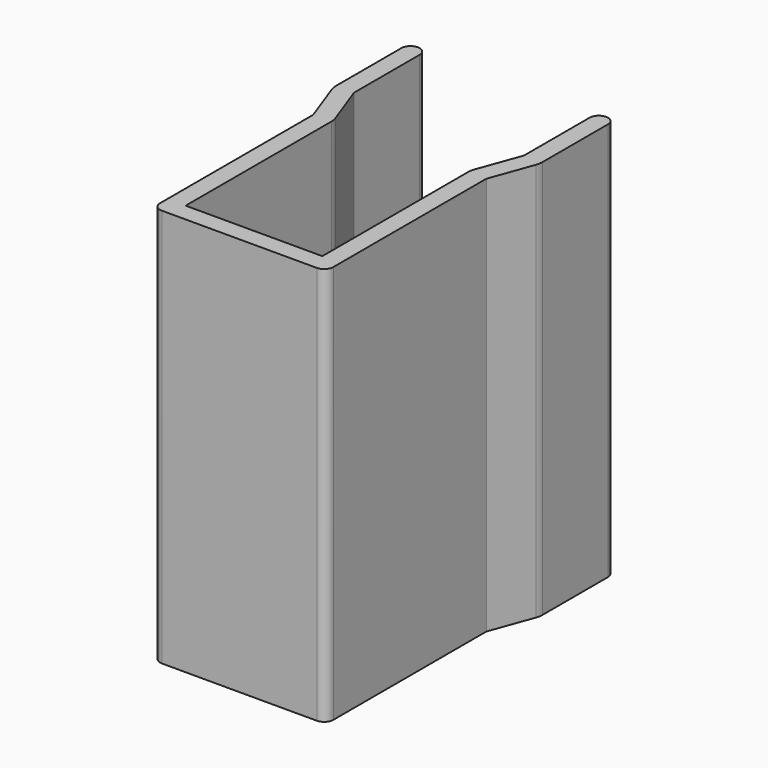
from build123d import *

# Parameters (mm, degrees)
F0_W     = 1.6
F0_H     = 8
F1_DEPTH = 35
F2_R     = 0.79999


# Not quite as in the source:
# - a fillet or chamfer is up to 0.001 mm smaller than in the source, because OpenCascade refuses the exact size


with BuildPart() as f1:
    # F0 (on Top) → F1 (new body)
    with BuildSketch(Plane.XY):
        Polygon((0, 16), (0, 0), (-12, 0), (-12, 16), (-13.6, 16), (-13.6, -1.6), (1.6, -1.6), (1.6, 16), align=None)
        with BuildLine():
            ThreePointArc((0.0964918067, 16.5472322293), (0.0243075952, 16.2778370843), (0, 16))
            Line((0, 16), (1.6, 16))
            Line((1.6, 16), (0.0964918067, 16.5472322293))
        make_face()
        with BuildLine():
            Line((-13.6, 16), (-12, 16))
            ThreePointArc((-12, 16), (-12.0243075952, 16.2778370843), (-12.0964918067, 16.5472322293))
            Line((-12.0964918067, 16.5472322293), (-13.6, 16))
        make_face()
        Polygon((0.0964918067, 16.5472322293), (1.6, 16), (2.9680805733, 19.7587704831), (1.46457238, 20.3060027125), align=None)
        Polygon((-14.9680805733, 19.7587704831), (-13.6, 16), (-12.0964918067, 16.5472322293), (-13.46457238, 20.3060027125), align=None)
        with BuildLine():
            Line((1.46457238, 20.3060027125), (2.9680805733, 19.7587704831))
            ThreePointArc((2.9680805733, 19.7587704831), (3.0402647849, 20.0281656282), (3.06457238, 20.3060027125))
            Line((3.06457238, 20.3060027125), (1.46457238, 20.3060027125))
        make_face()
        with Locations((2.26457238, 24.3060027125)):
            Rectangle(F0_W, F0_H)
        with BuildLine():
            ThreePointArc((-15.06457238, 20.3060027125), (-15.0402647849, 20.0281656282), (-14.9680805733, 19.7587704831))
            Line((-14.9680805733, 19.7587704831), (-13.46457238, 20.3060027125))
            Line((-13.46457238, 20.3060027125), (-15.06457238, 20.3060027125))
        make_face()
        with Locations((-14.26457238, 24.3060027125)):
            Rectangle(F0_W, F0_H)
    extrude(amount=F1_DEPTH)

    # F2 (radius 0.8 in the source; OpenCascade refuses exactly that, so slightly less here)
    f2_edges = [f1.edges().sort_by_distance(p)[0] for p in [
        (1.6, -1.6, 17.5),
        (-13.6, -1.6, 17.5),
        (-15.064572, 28.306003, 17.5),
        (3.064572, 28.306003, 17.5),
        (1.464572, 28.306003, 17.5),
        (-13.464572, 28.306003, 17.5),
    ]]
    fillet(f2_edges, radius=F2_R)


solid = f1.part
